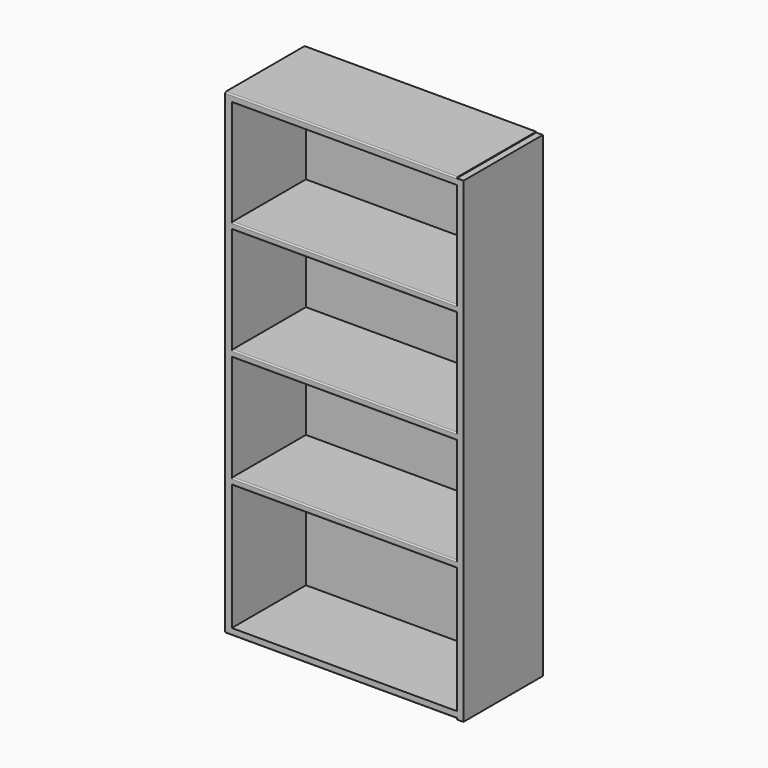
from build123d import *

# Parameters (mm, degrees)
F0_W     = 863.595354099
F0_H     = 25.4
F1_DEPTH = 381
F2_R     = 5.08
F0_H_2   = 482.6
F0_H_3   = 406.4
F3_DEPTH = 25.4


with BuildPart() as f1:
    # F0 (on Front) → F1 (new body)
    with BuildSketch(Plane.XZ):
        Polygon((-12.7, 891.914858846), (-12.7, 914.4), (-12.7, 917.314858846), (-876.295354099, 917.314858846), (-876.295354099, 891.914858846), align=None)
        with Locations((-444.4976770495, -898.785141154)):
            Rectangle(F0_W, F0_H)
        Polygon((-901.695354099, -911.485141154), (-876.295354099, -911.485141154), (-876.295354099, -886.085141154), (-876.295354099, -403.485141154), (-876.295354099, -378.085141154), (-876.295354099, 28.314858846), (-876.295354099, 53.714858846), (-876.295354099, 460.114858846), (-876.295354099, 485.514858846), (-876.295354099, 891.914858846), (-876.295354099, 917.314858846), (-901.695354099, 917.314858846), align=None)
        Polygon((-12.7, -911.485141154), (-12.7, -914.4), (12.7, -914.4), (12.7, 914.4), (-12.7, 914.4), (-12.7, 891.914858846), (-12.7, 485.514858846), (-12.7, 460.114858846), (-12.7, 53.714858846), (-12.7, 28.314858846), (-12.7, -378.085141154), (-12.7, -403.485141154), (-12.7, -886.085141154), align=None)
        with Locations((-444.4976770495, 472.814858846)):
            Rectangle(F0_W, F0_H)
        with Locations((-444.4976770495, 41.014858846)):
            Rectangle(F0_W, F0_H)
        with Locations((-444.4976770495, -390.785141154)):
            Rectangle(F0_W, F0_H)
    extrude(amount=F1_DEPTH)

    # F2
    f2_edges = [f1.edges().sort_by_distance(p)[0] for p in [
        (-457.197677, -381, 917.314859),
        (-444.497677, -381, 485.514859),
        (-444.497677, -381, 460.114859),
        (-444.497677, -381, 53.714859),
        (-444.497677, -381, -378.085141),
        (-444.497677, -381, 28.314859),
        (-444.497677, -381, -403.485141),
        (-457.197677, -381, -911.485141),
    ]]
    fillet(f2_edges, radius=F2_R)

    # F0 (on Front) → F3 (join)
    with BuildSketch(Plane.XZ):
        with Locations((-444.4976770495, -644.785141154)):
            Rectangle(F0_W, F0_H_2)
        with Locations((-444.4976770495, -174.885141154)):
            Rectangle(F0_W, F0_H_3)
        with Locations((-444.4976770495, 256.914858846)):
            Rectangle(F0_W, F0_H_3)
        with Locations((-444.4976770495, 688.714858846)):
            Rectangle(F0_W, F0_H_3)
    extrude(amount=F3_DEPTH)


solid = f1.part
